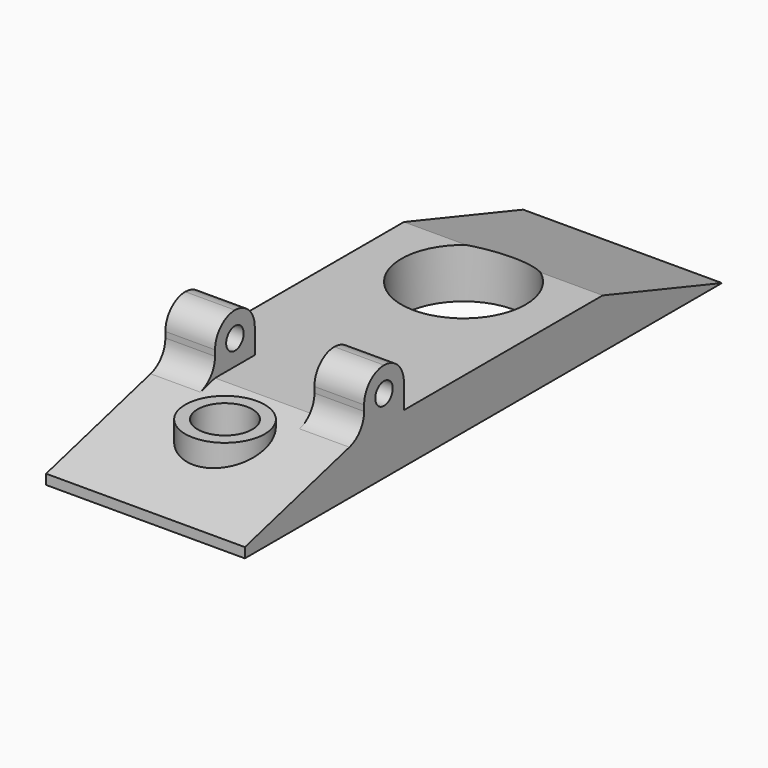
from build123d import *

# Parameters (mm, degrees)
F0_W         = 20
F0_H         = 60
F0_R         = 4
F0_R_2       = 6.25
F1_DEPTH     = 4
F1_FACE_W    = 20
F1_FACE_H    = 60
F1_FACE_R    = 4
F1_FACE_R_2  = 6.25
F0_R_3       = 2.75
F2_DEPTH     = 1
F3_W         = 5
F3_H         = 5
F4_DEPTH     = 5
F5_T1_DEPTH  = 97.9025398997
F6_R         = 2.49999
F7_R         = 1.1
F8_DEPTH     = 25
F9_DEPTH     = 5
F10_T1_DEPTH = 97.8518303197
F11_DEPTH    = 2


# Not quite as in the source:
# - a fillet or chamfer that OpenCascade refuses, or shapes differently, is made with other operations: its cross-section is extruded or revolved along the edge and cut away or added
# - a fillet or chamfer is up to 0.001 mm smaller than in the source, because OpenCascade refuses the exact size


with BuildPart() as f1:
    # F0 (on Top) → F1 (new body)
    with BuildSketch(Plane.XY):
        with Locations((10, 30)):
            Rectangle(F0_W, F0_H)
        with Locations((10, 10)):
            Circle(F0_R, mode=Mode.SUBTRACT)
        with Locations((10, 40)):
            Circle(F0_R_2, mode=Mode.SUBTRACT)
    extrude(amount=F1_DEPTH)

    # F1_face (on face) + F0 (on Top) → F2 (join)
    with BuildSketch(Plane(origin=(10, 29.783961526, 4), x_dir=(1, 0, 0), z_dir=(0, 0, 1))):
        with Locations((0, 0.216038474)):
            Rectangle(F1_FACE_W, F1_FACE_H)
        with Locations((0, -19.783961526)):
            Circle(F1_FACE_R, mode=Mode.SUBTRACT)
        with Locations((0, 10.216038474)):
            Circle(F1_FACE_R_2, mode=Mode.SUBTRACT)
    with BuildSketch(Plane.XY):
        with Locations((10, 10)):
            Circle(F0_R)
        with Locations((10, 10)):
            Circle(F0_R_3, mode=Mode.SUBTRACT)
    extrude(amount=F2_DEPTH)

    # F3 (on face) → F4 (join)
    with BuildSketch(Plane.XY.offset(5)):
        with Locations((2.5, 17.5)):
            Rectangle(F3_W, F3_H)
        with Locations((17.5, 17.5)):
            Rectangle(F3_W, F3_H)
    extrude(amount=F4_DEPTH)

    # F5: chamfer of 15 x 4 on 1 edges, made by hand

    # F5_s2 → F5_t1 (cut)
    with BuildSketch(Plane.YZ.offset(-38.9512699498)):
        Polygon((15, 5), (0, 1), (0, 5), align=None)
    extrude(amount=F5_T1_DEPTH, mode=Mode.SUBTRACT)

    # F6 (radius 2.5 in the source; OpenCascade refuses exactly that, so slightly less here)
    f6_edges = [f1.edges().sort_by_distance(p)[0] for p in [
        (2.5, 15, 5),
        (2.5, 15, 10),
        (17.5, 15, 5),
        (17.5, 15, 10),
        (2.5, 20, 10),
        (17.5, 20, 10),
    ]]
    fillet(f6_edges, radius=F6_R)

    # F7 (on face) → F8 (cut)
    with BuildSketch(Plane(origin=(0, 0, 0), x_dir=(0, -1, 0), z_dir=(-1, 0, 0))):
        with Locations((-17.5, 7.5)):
            Circle(F7_R)
    extrude(amount=-F8_DEPTH, mode=Mode.SUBTRACT)

    # F10: chamfer of 5 x 15 on 1 edges, made by hand

    # F10_s2 → F10_t1 (cut)
    with BuildSketch(Plane.YZ.offset(-38.9259151598)):
        Polygon((60, 0), (45, 5), (60, 5), align=None)
    extrude(amount=F10_T1_DEPTH, mode=Mode.SUBTRACT)



with BuildPart() as f9:
    # F0 (on Top) → F9 (new body)
    with BuildSketch(Plane.XY):
        with Locations((10, 10)):
            Circle(F0_R)
        with Locations((10, 10)):
            Circle(F0_R_3, mode=Mode.SUBTRACT)
    extrude(amount=F9_DEPTH)


with BuildPart() as f1_1:
    add(f1.part)

    add(f9.part)  # F11 merges F9
    # F0 (on Top) → F11 (join)
    with BuildSketch(Plane.XY):
        with Locations((10, 10)):
            Circle(F0_R_3)
    extrude(amount=F11_DEPTH)


solid = f1_1.part
